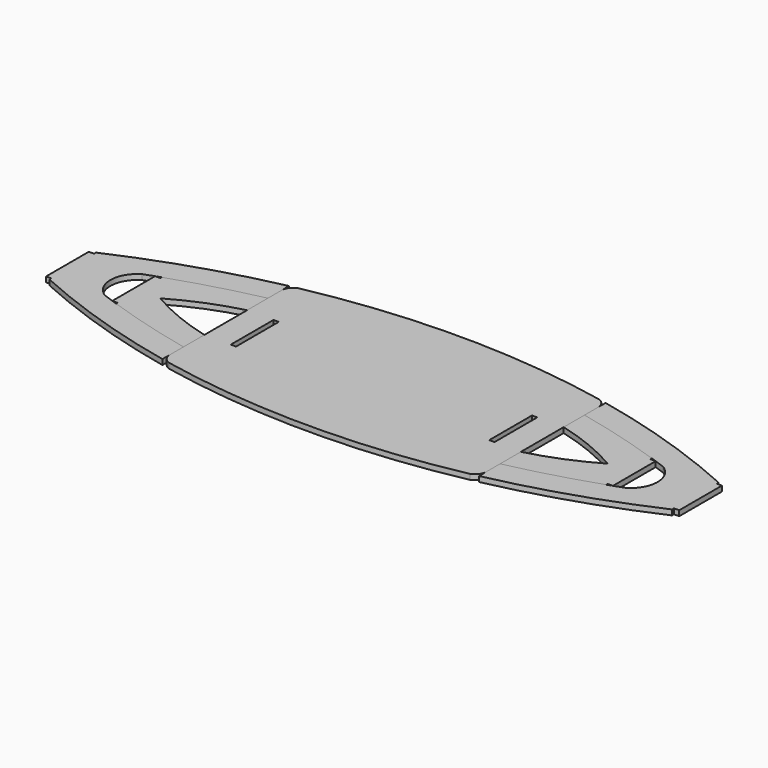
from build123d import *

# Parameters (mm, degrees)
F1_DEPTH = 10
F0_W     = 10
F0_H     = 101.2735754151
F2_DEPTH = 10
F3_DEPTH = 10


with BuildPart() as f1:
    # F0 (on Top) → F1 (new body)
    with BuildSketch(Plane.XY):
        with BuildLine():
            ThreePointArc((590, 55.1744807956), (447.5186809208, 110.2899924962), (300, 150))
            Line((300, 150), (300, 133.7422728539))
            Line((300, 133.7422728539), (300, 100))
            ThreePointArc((300, 100), (382.9034698068, 79.4411893647), (464.4737208674, 54.104572727))
            ThreePointArc((464.4737208674, 54.104572727), (469.476840252, 52.3796755402), (474.4737208674, 50.6367877075))
            ThreePointArc((474.4737208674, 50.6367877075), (484.624267711, 48.1306176712), (494.0528874295, 43.612252958))
            ThreePointArc((494.0528874295, 43.612252958), (547.4512685754, 22.8381522122), (600, 0))
            Line((600, 0), (600, 50.6367877075))
            Line((600, 50.6367877075), (590, 50.6367877075))
            Line((590, 50.6367877075), (590, 55.1744807956))
        make_face()
        with BuildLine():
            ThreePointArc((494.0528874295, -43.612252958), (547.4512685754, -22.8381522122), (600, 0))
            ThreePointArc((600, 0), (547.4512685754, 22.8381522122), (494.0528874295, 43.612252958))
            ThreePointArc((494.0528874295, 43.612252958), (518.4907252716, 0), (494.0528874295, -43.612252958))
        make_face()
        with BuildLine():
            Line((600, -50.6367877075), (600, 0))
            ThreePointArc((600, 0), (547.4512685754, -22.8381522122), (494.0528874295, -43.612252958))
            ThreePointArc((494.0528874295, -43.612252958), (484.624267711, -48.1306176712), (474.4737208674, -50.6367877075))
            ThreePointArc((474.4737208674, -50.6367877075), (469.476840252, -52.3796755402), (464.4737208674, -54.104572727))
            ThreePointArc((464.4737208674, -54.104572727), (382.9034698068, -79.4411893647), (300, -100))
            Line((300, -100), (300, -133.7422728539))
            Line((300, -133.7422728539), (300, -150))
            ThreePointArc((300, -150), (447.5186809208, -110.2899924962), (590, -55.1744807956))
            Line((590, -55.1744807956), (590, -50.6367877075))
            Line((590, -50.6367877075), (600, -50.6367877075))
        make_face()
        with BuildLine():
            ThreePointArc((494.0528874295, 43.612252958), (484.624267711, 48.1306176712), (474.4737208674, 50.6367877075))
            ThreePointArc((474.4737208674, 50.6367877075), (484.2757225927, 47.1591336982), (494.0528874295, 43.612252958))
        make_face()
        with BuildLine():
            ThreePointArc((474.4737208674, -50.6367877075), (484.624267711, -48.1306176712), (494.0528874295, -43.612252958))
            ThreePointArc((494.0528874295, -43.612252958), (484.2757225927, -47.1591336982), (474.4737208674, -50.6367877075))
        make_face()
    extrude(amount=F1_DEPTH)


with BuildPart() as f1b:
    # F0 (on Top) → F1, piece 2 (new body)
    with BuildSketch(Plane.XY):
        with BuildLine():
            Line((-300, 133.7422728539), (-300, 150))
            ThreePointArc((-300, 150), (-447.5186809208, 110.2899924962), (-590, 55.1744807956))
            Line((-590, 55.1744807956), (-590, 50.6367877075))
            Line((-590, 50.6367877075), (-600, 50.6367877075))
            Line((-600, 50.6367877075), (-600, 0))
            ThreePointArc((-600, 0), (-547.4512685754, 22.8381522122), (-494.0528874295, 43.612252958))
            ThreePointArc((-494.0528874295, 43.612252958), (-484.624267711, 48.1306176712), (-474.4737208674, 50.6367877075))
            ThreePointArc((-474.4737208674, 50.6367877075), (-469.476840252, 52.3796755402), (-464.4737208674, 54.104572727))
            ThreePointArc((-464.4737208674, 54.104572727), (-382.9034698068, 79.4411893647), (-300, 100))
            Line((-300, 100), (-300, 133.7422728539))
        make_face()
        with BuildLine():
            Line((-600, 0), (-600, -50.6367877075))
            Line((-600, -50.6367877075), (-590, -50.6367877075))
            Line((-590, -50.6367877075), (-590, -55.1744807956))
            ThreePointArc((-590, -55.1744807956), (-447.5186809208, -110.2899924962), (-300, -150))
            Line((-300, -150), (-300, -133.7422728539))
            Line((-300, -133.7422728539), (-300, -100))
            ThreePointArc((-300, -100), (-382.9034698068, -79.4411893647), (-464.4737208674, -54.104572727))
            ThreePointArc((-464.4737208674, -54.104572727), (-469.476840252, -52.3796755402), (-474.4737208674, -50.6367877075))
            ThreePointArc((-474.4737208674, -50.6367877075), (-484.624267711, -48.1306176712), (-494.0528874295, -43.612252958))
            ThreePointArc((-494.0528874295, -43.612252958), (-547.4512685754, -22.8381522122), (-600, 0))
        make_face()
        with BuildLine():
            ThreePointArc((-494.0528874295, 43.612252958), (-547.4512685754, 22.8381522122), (-600, 0))
            ThreePointArc((-600, 0), (-547.4512685754, -22.8381522122), (-494.0528874295, -43.612252958))
            ThreePointArc((-494.0528874295, -43.612252958), (-518.4907252716, 0), (-494.0528874295, 43.612252958))
        make_face()
        with BuildLine():
            ThreePointArc((-494.0528874295, 43.612252958), (-484.2757225927, 47.1591336982), (-474.4737208674, 50.6367877075))
            ThreePointArc((-474.4737208674, 50.6367877075), (-484.624267711, 48.1306176712), (-494.0528874295, 43.612252958))
        make_face()
        with BuildLine():
            ThreePointArc((-474.4737208674, -50.6367877075), (-484.2757225927, -47.1591336982), (-494.0528874295, -43.612252958))
            ThreePointArc((-494.0528874295, -43.612252958), (-484.624267711, -48.1306176712), (-474.4737208674, -50.6367877075))
        make_face()
    extrude(amount=F1_DEPTH)


with BuildPart() as f2:
    # F0 (on Top) → F2 (new body)
    with BuildSketch(Plane.XY):
        with BuildLine():
            Line((300, 100), (300, 133.7422728539))
            ThreePointArc((300, 133.7422728539), (295.4955610638, 145.4649254676), (285.4628431703, 153.0184098359))
            ThreePointArc((285.4628431703, 153.0184098359), (0, 181.5981851), (-285.4628431703, 153.0184098359))
            ThreePointArc((-285.4628431703, 153.0184098359), (-295.4955610638, 145.4649254676), (-300, 133.7422728539))
            Line((-300, 133.7422728539), (-300, 100))
            Line((-300, 100), (-300, 50.6367877075))
            Line((-300, 50.6367877075), (-300, -50.6367877075))
            Line((-300, -50.6367877075), (-300, -100))
            Line((-300, -100), (-300, -133.7422728539))
            ThreePointArc((-300, -133.7422728539), (-295.4955610638, -145.4649254676), (-285.4628431703, -153.0184098359))
            ThreePointArc((-285.4628431703, -153.0184098359), (0, -181.5981851), (285.4628431703, -153.0184098359))
            ThreePointArc((285.4628431703, -153.0184098359), (295.4955610638, -145.4649254676), (300, -133.7422728539))
            Line((300, -133.7422728539), (300, -100))
            Line((300, -100), (300, -50.6367877075))
            Line((300, -50.6367877075), (300, 50.6367877075))
            Line((300, 50.6367877075), (300, 100))
        make_face()
        with Locations((-245, 0)):
            Rectangle(F0_W, F0_H, mode=Mode.SUBTRACT)
        with Locations((245, 0)):
            Rectangle(F0_W, F0_H, mode=Mode.SUBTRACT)
    extrude(amount=F2_DEPTH)


with BuildPart() as f3:
    # F0 (on Top) → F3 (new body)
    with BuildSketch(Plane.XY):
        with BuildLine():
            Line((-300, 50.6367877075), (-300, 100))
            ThreePointArc((-300, 100), (-382.9034698068, 79.4411893647), (-464.4737208674, 54.104572727))
            Line((-464.4737208674, 54.104572727), (-464.4737208674, 50.6367877075))
            Line((-464.4737208674, 50.6367877075), (-474.4737208674, 50.6367877075))
            Line((-474.4737208674, 50.6367877075), (-474.4737208674, -50.6367877075))
            Line((-474.4737208674, -50.6367877075), (-464.4737208674, -50.6367877075))
            Line((-464.4737208674, -50.6367877075), (-464.4737208674, -54.104572727))
            ThreePointArc((-464.4737208674, -54.104572727), (-382.9034698068, -79.4411893647), (-300, -100))
            Line((-300, -100), (-300, -50.6367877075))
            ThreePointArc((-300, -50.6367877075), (-363.754185083, -29.5472367405), (-424.0561425686, 0))
            ThreePointArc((-424.0561425686, 0), (-363.754185083, 29.5472367405), (-300, 50.6367877075))
        make_face()
    extrude(amount=F3_DEPTH)


with BuildPart() as f3b:
    # F0 (on Top) → F3, piece 2 (new body)
    with BuildSketch(Plane.XY):
        with BuildLine():
            ThreePointArc((464.4737208674, 54.104572727), (382.9034698068, 79.4411893647), (300, 100))
            Line((300, 100), (300, 50.6367877075))
            ThreePointArc((300, 50.6367877075), (363.754185083, 29.5472367405), (424.0561425686, 0))
            ThreePointArc((424.0561425686, 0), (363.754185083, -29.5472367405), (300, -50.6367877075))
            Line((300, -50.6367877075), (300, -100))
            ThreePointArc((300, -100), (382.9034698068, -79.4411893647), (464.4737208674, -54.104572727))
            Line((464.4737208674, -54.104572727), (464.4737208674, -50.6367877075))
            Line((464.4737208674, -50.6367877075), (474.4737208674, -50.6367877075))
            Line((474.4737208674, -50.6367877075), (474.4737208674, 50.6367877075))
            Line((474.4737208674, 50.6367877075), (464.4737208674, 50.6367877075))
            Line((464.4737208674, 50.6367877075), (464.4737208674, 54.104572727))
        make_face()
    extrude(amount=F3_DEPTH)


solid = Compound([f1.part, f1b.part, f2.part, f3.part, f3b.part])
